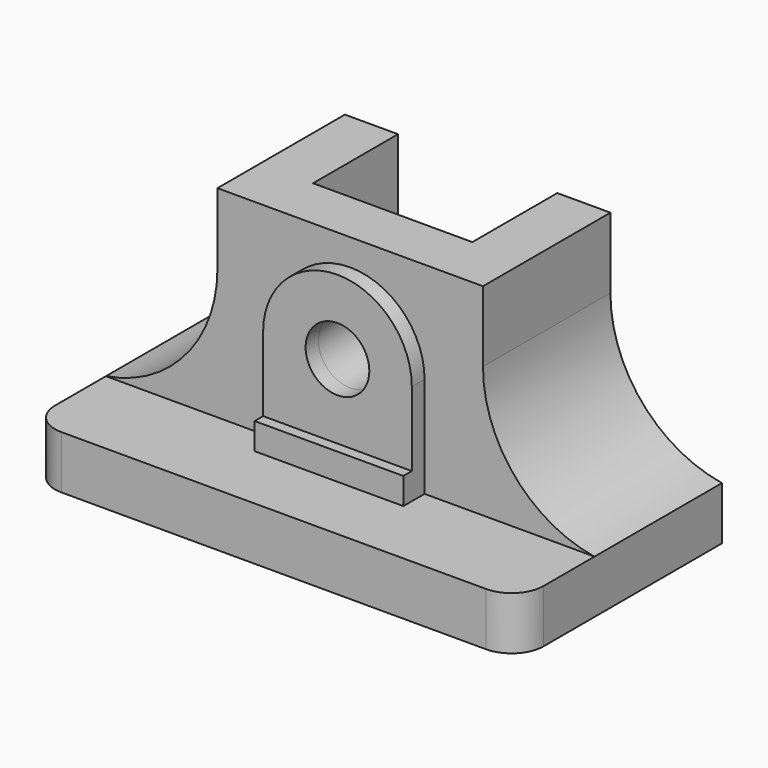
from build123d import *

# Parameters (mm, degrees)
F1_DEPTH    = 10
F3_DEPTH    = 48
F4_T1_DEPTH = 30
F5_T1_DEPTH = 30
F6_R        = 6
F7_DEPTH    = 3
F8_W        = 28
F8_H        = 5
F9_DEPTH    = 2
F10_DEPTH   = 25


# Not quite as in the source:
# - a fillet or chamfer that OpenCascade refuses, or shapes differently, is made with other operations: its cross-section is extruded or revolved along the edge and cut away or added


with BuildPart() as f1:
    # F0 (on Top) → F1 (new body)
    with BuildSketch(Plane.XY):
        with BuildLine():
            Line((-15, 30), (-46, 30))
            Line((-46, 30), (-46, -12))
            ThreePointArc((-46, -12), (-44.2426406871, -16.2426406871), (-40, -18))
            Line((-40, -18), (40, -18))
            ThreePointArc((40, -18), (44.2426406871, -16.2426406871), (46, -12))
            Line((46, -12), (46, 30))
            Line((46, 30), (15, 30))
            Line((15, 30), (15, 10))
            Line((15, 10), (-15, 10))
            Line((-15, 10), (-15, 30))
        make_face()
    extrude(amount=F1_DEPTH)

    # F2 (on Top) → F3 (join)
    with BuildSketch(Plane.XY):
        Polygon((-15, 30), (-25, 30), (-25, 0), (25, 0), (25, 30), (15, 30), (15, 10), (-15, 10), align=None)
    extrude(amount=F3_DEPTH)

    # F4: fillet of radius 25 on 1 edges, made by hand

    # F4_s2 → F4_t1 (join)
    with BuildSketch(Plane.XZ.offset(-30)):
        with BuildLine():
            ThreePointArc((-46, 10), (-30.9605672353, 18.4760736125), (-25, 34.6779253585))
            Line((-25, 34.6779253585), (-25, 10))
            Line((-25, 10), (-46, 10))
        make_face()
    extrude(amount=F4_T1_DEPTH)

    # F5: fillet of radius 25 on 1 edges, made by hand

    # F5_s2 → F5_t1 (join)
    with BuildSketch(Plane.XZ.offset(-30)):
        with BuildLine():
            ThreePointArc((46, 10), (30.9605672353, 18.4760736125), (25, 34.6779253585))
            Line((25, 34.6779253585), (25, 10))
            Line((25, 10), (46, 10))
        make_face()
    extrude(amount=F5_T1_DEPTH)

    # F6 (on face) → F7 (join)
    with BuildSketch(Plane.XZ):
        with BuildLine():
            Line((14, 10), (14, 29))
            ThreePointArc((14, 29), (0, 43), (-14, 29))
            Line((-14, 29), (-14, 10))
            Line((-14, 10), (14, 10))
        make_face()
        with Locations((0, 29)):
            Circle(F6_R, mode=Mode.SUBTRACT)
    extrude(amount=F7_DEPTH)

    # F8 (on face) → F9 (join)
    with BuildSketch(Plane.XZ.offset(3)):
        with Locations((0, 12.5)):
            Rectangle(F8_W, F8_H)
    extrude(amount=F9_DEPTH)

    # F10 (cut): a face of the model
    f10_faces = [f1.faces().sort_by_distance(p)[0] for p in [
        (0, 0, 29),
    ]]
    extrude(f10_faces, amount=-F10_DEPTH, mode=Mode.SUBTRACT)


solid = f1.part
